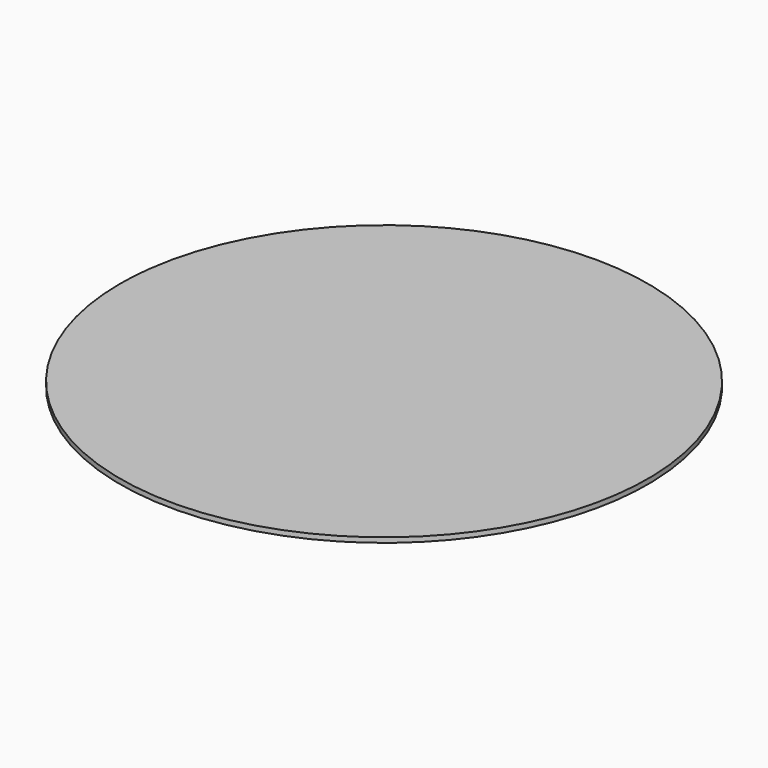
from build123d import *

# Parameters (mm, degrees)
F1_DEPTH = 1


# Not quite as in the source:
# - a feature names something its author has since deleted; it is built from what else it names


with BuildPart() as f1:
    # F0 (on Top) → F1 (new body)
    with BuildSketch(Plane.XY):
        with BuildLine():
            add(Edge.make_bspline(
                [(-53.5, 0), (-53.5, -92.6647182049), (26.75, -46.3323591025), (107, 0), (26.75, 46.3323591025), (-53.5, 92.6647182049), (-53.5, 0)],
                knots=[0, 0, 0, 2.0943951024, 2.0943951024, 4.1887902048, 4.1887902048, 6.2831853072, 6.2831853072, 6.2831853072], degree=2, weights=[1, 0.5, 1, 0.5, 1, 0.5, 1]))
        make_face()
    extrude(amount=F1_DEPTH)


solid = f1.part
